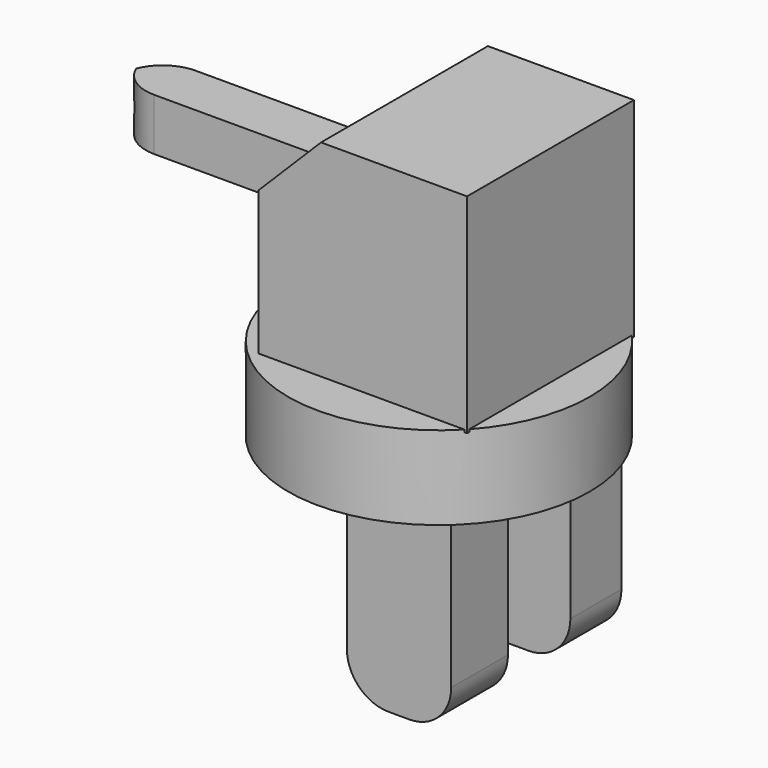
from build123d import *

# Parameters (mm, degrees)
F1_DEPTH     = 12.7
F0_W         = 25.4
F0_H         = 6.35
F2_DEPTH     = 3.175
F3_SIZE      = 7.62
F4_R         = 18.3677824361
F5_DEPTH     = 10.16
F6_W         = 8.6341705173
F6_H         = 22.7366536856
F6_W_2       = 7.7707553282
F7_DEPTH     = 12.7
F8_R         = 5.08
F9_R         = 1.736345134
F10_DEPTH    = 177.8
F11_T1_DEPTH = 31.75
F12_W        = 3.81
F12_H        = 3.810003606
F12_H_2      = 3.81
F13_DEPTH    = 25.4


# Not quite as in the source:
# - a fillet or chamfer that OpenCascade refuses, or shapes differently, is made with other operations: its cross-section is extruded or revolved along the edge and cut away or added


with BuildPart() as f1:
    # F0 (on Front) → F1 (new body, symmetric)
    with BuildSketch(Plane.XZ):
        Polygon((1.495771724, 35.256898239), (-23.904228276, 35.256898239), (-23.904228276, 27.4009877652), (-23.904228276, 21.0509877652), (-23.904228276, 9.856898239), (1.495771724, 9.856898239), align=None)
    extrude(amount=F1_DEPTH, both=True)

    # F0 (on Front) → F2 (join, symmetric)
    with BuildSketch(Plane.XZ):
        with Locations((-36.604228276, 24.2259877652)):
            Rectangle(F0_W, F0_H)
    extrude(amount=F2_DEPTH, both=True)

    # F3
    f3_edges = [f1.edges().sort_by_distance(p)[0] for p in [
        (-23.904228, 0, 35.256898),
    ]]
    chamfer(f3_edges, length=F3_SIZE)

    # F4 (on Top) → F5 (join)
    with BuildSketch(Plane.XY):
        with Locations((-12.0878415182, 0)):
            Circle(F4_R)
    extrude(amount=F5_DEPTH)

    # F6 (on Right) → F7 (join)
    with BuildSketch(Plane.YZ):
        with Locations((-8.9219780639, -11.3683268428)):
            Rectangle(F6_W, F6_H)
        with Locations((8.7780752219, -11.3683268428)):
            Rectangle(F6_W_2, F6_H)
    extrude(amount=-F7_DEPTH)

    # F8
    f8_edges = [f1.edges().sort_by_distance(p)[0] for p in [
        (-12.7, 8.778075, -22.736654),
        (-12.7, -8.921978, -22.736654),
        (0, -8.921978, -22.736654),
        (0, 8.778075, -22.736654),
    ]]
    fillet(f8_edges, radius=F8_R)

    # F9 (on Right) → F10 (cut)
    with BuildSketch(Plane.YZ):
        with Locations((0, 24.2223944515)):
            Circle(F9_R)
    extrude(amount=-F10_DEPTH, mode=Mode.SUBTRACT)

    # F11: fillet of radius 5.08 on 2 edges, made by hand

    # F11_s2 → F11_t1 (cut)
    with BuildSketch(Plane.XY.offset(8.3509877652)):
        with BuildLine():
            ThreePointArc((-44.224228276, 3.175), (-47.8163307244, 1.6871024484), (-49.304228276, -1.905))
            Line((-49.304228276, -1.905), (-49.304228276, 3.175))
            Line((-49.304228276, 3.175), (-44.224228276, 3.175))
        make_face()
        with BuildLine():
            ThreePointArc((-44.224228276, -3.175), (-47.8163307244, -1.6871024484), (-49.304228276, 1.905))
            Line((-49.304228276, 1.905), (-49.304228276, -3.175))
            Line((-49.304228276, -3.175), (-44.224228276, -3.175))
        make_face()
    extrude(amount=F11_T1_DEPTH, mode=Mode.SUBTRACT)

    # F12 (on Right) → F13 (cut)
    with BuildSketch(Plane.YZ):
        with Locations((7.1409824217, 30.2377566695)):
            Rectangle(F12_W, F12_H)
        with Locations((-8.4303260025, 30.2377548665)):
            Rectangle(F12_W, F12_H_2)
    extrude(amount=-F13_DEPTH, mode=Mode.SUBTRACT)


solid = f1.part
